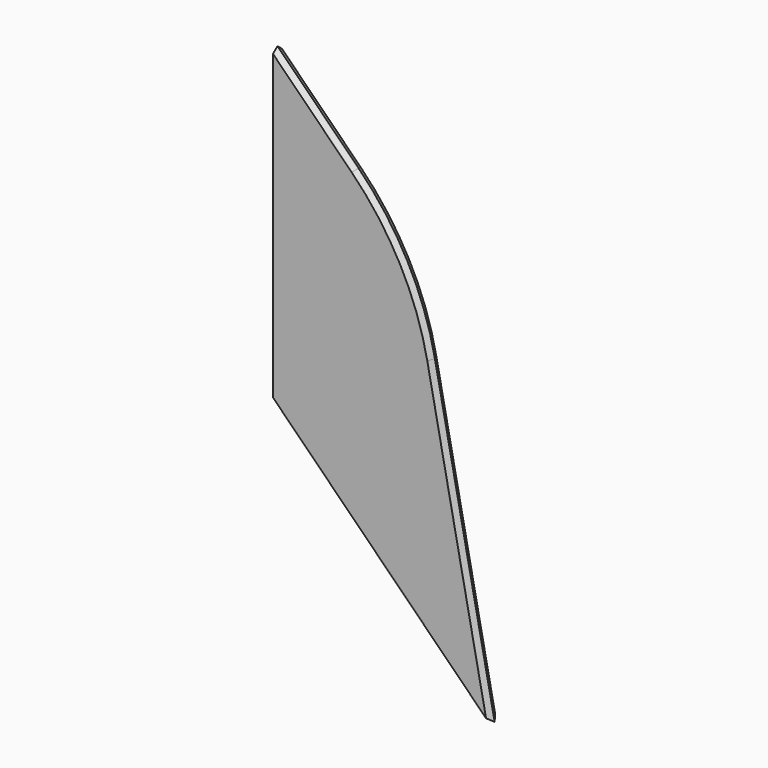
from build123d import *

# Parameters (mm, degrees)
F1_DEPTH = 2
F2_R     = 50
F3_SIZE2 = 0.57734
F3_SIZE  = 0.99999


# Not quite as in the source:
# - a fillet or chamfer is up to 0.001 mm smaller than in the source, because OpenCascade refuses the exact size


with BuildPart() as f1:
    # F0 (on Front) → F1 (new body)
    with BuildSketch(Plane.XZ):
        Polygon((0, 55), (0, 0), (38.8908729653, -38.8908729653), (25.2356788824, 29.7643211176), align=None)
    extrude(amount=F1_DEPTH)

    # F2
    f2_edges = [f1.edges().sort_by_distance(p)[0] for p in [
        (25.235679, -1, 29.764321),
    ]]
    fillet(f2_edges, radius=F2_R)

    # F3 (size 1 and 0.5773502692 in the source; OpenCascade refuses exactly that, so slightly less here)
    f3_edges = [f1.edges().sort_by_distance(p)[0] for p in [
        (7.255218, -2, 47.744782),
        (7.255218, 0, 47.744782),
    ]]
    f3_side = f1.faces().sort_by_distance((7.255218, -1, 47.744782))[0]
    chamfer(f3_edges, length=F3_SIZE, length2=F3_SIZE2, reference=f3_side)


solid = f1.part
